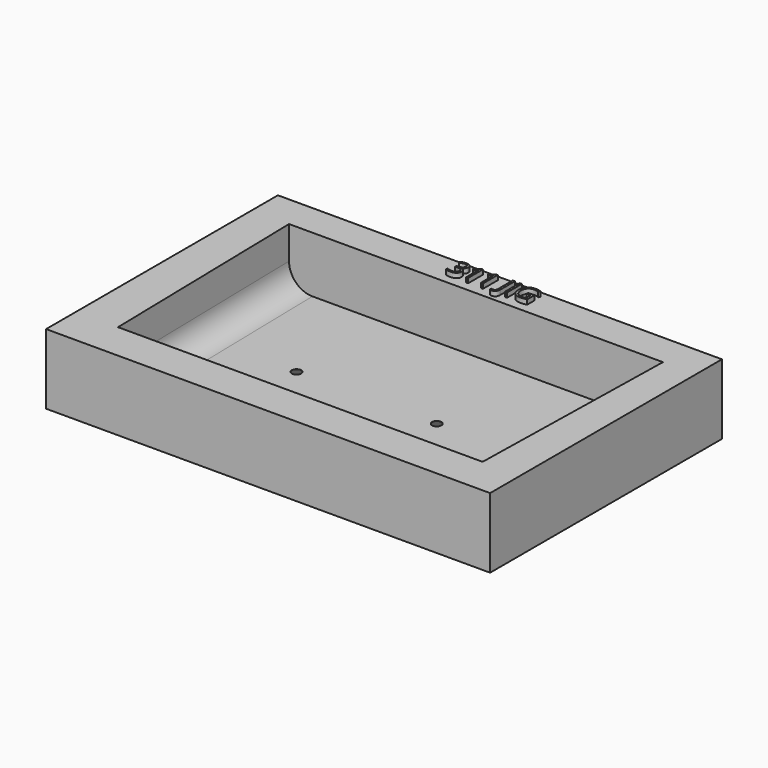
from build123d import *

# Parameters (mm, degrees)
F1_W           = 95
F1_H           = 62
F2_DEPTH       = 15
F0_W           = 95
F0_H           = 62
F3_DEPTH       = 3
F5_D           = 2
F5_CSINK_D     = 7
F5_CSINK_ANGLE = 80
F6_R           = 5
F7_R           = 5
F8_TEXT_SIZE   = 5.5618170235
F9_DEPTH       = 1


# Not quite as in the source:
# - Text() gives the source's letters only with a copy of the font that has no kerning and outlines rounded to 1/6400 em; it was checked with that copy


with BuildPart() as f2:
    # F1 (on face) → F2 (new body)
    with BuildSketch(Plane.XY):
        Rectangle(F1_W, F1_H)
        Polygon((-38.5472966552, -22.9523805958), (-39.5472966552, 24.036979902), (40.4527033448, 24.036979902), (39.4527033448, -22.9523805958), align=None, mode=Mode.SUBTRACT)
    extrude(amount=F2_DEPTH)

    # F0 (on Top) → F3 (join)
    with BuildSketch(Plane.XY):
        Rectangle(F0_W, F0_H)
    extrude(amount=F3_DEPTH)

    # F5 (through all)
    with Locations(Plane(origin=(0, 0, 0), x_dir=(1, 0, 0), z_dir=(0, 0, -1))):
        with Locations((10.4522837698, -1.0369799566), (-19.5477162302, -1.0369799566)):
            CounterSinkHole(F5_D / 2, F5_CSINK_D / 2, counter_sink_angle=F5_CSINK_ANGLE)

    # F6
    f6_edges = [f2.edges().sort_by_distance(p)[0] for p in [
        (-39.047297, 0.5423, 3),
    ]]
    fillet(f6_edges, radius=F6_R)

    # F7
    f7_edges = [f2.edges().sort_by_distance(p)[0] for p in [
        (39.952703, 0.5423, 3),
    ]]
    fillet(f7_edges, radius=F7_R)

    # F8 (on face) → F9 (join)
    with BuildSketch(Plane.XY.offset(15)):
        with Locations((-7.9062916338, 25.9632784873)):
            Text('311 JIG', F8_TEXT_SIZE, font='Open Sans', text_align=(TextAlign.LEFT, TextAlign.BOTTOM))
    extrude(amount=F9_DEPTH)


solid = f2.part
